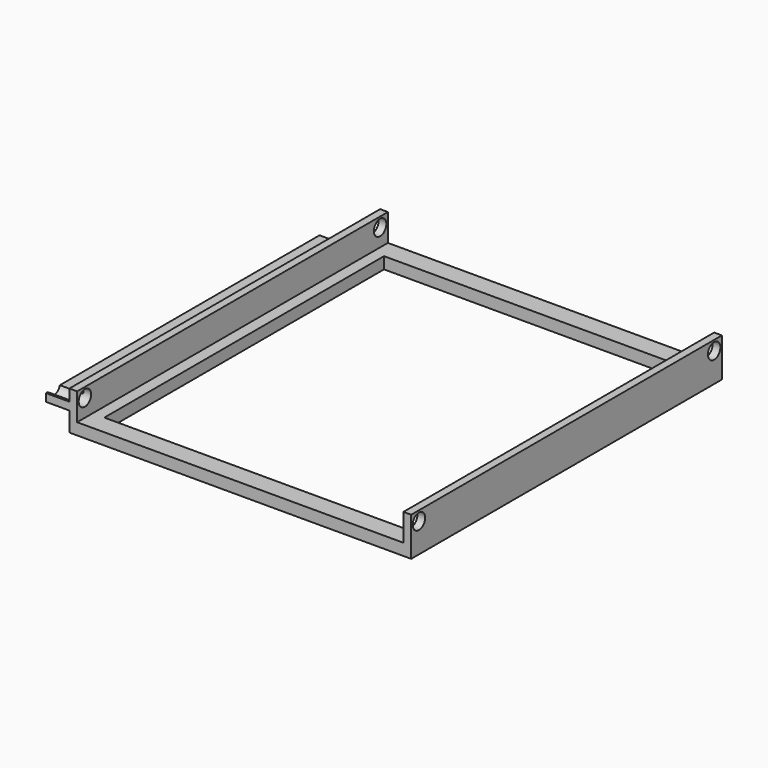
from build123d import *

# Parameters (mm, degrees)
F0_W      = 2
F0_H      = 3
F1_DEPTH  = 100
F2_W      = 78
F2_H      = 90
F1_FACE_W = 6
F1_FACE_H = 100
F3_DEPTH  = 3
F4_W      = 6
F4_H      = 12
F5_DEPTH  = 10
F7_D      = 4
F7_DEPTH  = 8.001
F9_D      = 4


# Not quite as in the source:
# - a feature names something its author has since deleted; it is built from what else it names


with BuildPart() as f1:
    # F0 (on Front) → F1 (new body)
    with BuildSketch(Plane.XZ):
        Polygon((-2, 0), (0, 0), (86, 0), (86, 10), (84, 10), (84, 3), (0, 3), (0, 7), (-2, 7), (-8, 7), (-8, 5), (-2, 5), align=None)
        with Locations((-1, 8.5)):
            Rectangle(F0_W, F0_H)
    extrude(amount=F1_DEPTH)

    # F2 (on Top) + F1_face (on face) → F3 (cut)
    with BuildSketch(Plane.XY):
        with Locations((42, -50)):
            Rectangle(F2_W, F2_H)
    with BuildSketch(Plane(origin=(-5, -50, 7), x_dir=(1, 0, 0), z_dir=(0, 0, 1))):
        Rectangle(F1_FACE_W, F1_FACE_H)
    extrude(amount=F3_DEPTH, mode=Mode.SUBTRACT)

    # F4 (on Top) → F5 (cut)
    with BuildSketch(Plane.XY):
        with Locations((-5, -6)):
            Rectangle(F4_W, F4_H)
    extrude(amount=F5_DEPTH, mode=Mode.SUBTRACT)

    # F7 (through all, one way)
    with BuildSketch(Plane.YZ):
        with Locations((-2.5, 7.5), (-97.5, 7.5)):
            Circle(F7_D / 2)
    extrude(amount=-F7_DEPTH, mode=Mode.SUBTRACT)

    # F9 (through all)
    with Locations(Plane(origin=(0, 0, 0), x_dir=(0, 1, 0), z_dir=(-1, 0, 0))):
        with Locations((-2.5, -7.5), (-97.5, -7.5)):
            Hole(F9_D / 2)


solid = f1.part
